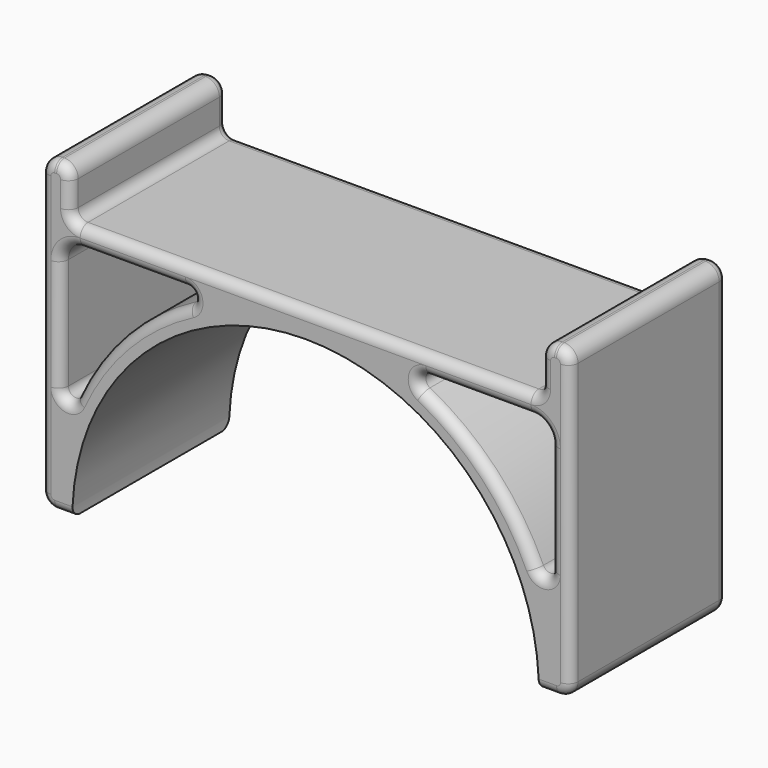
from build123d import *

# Parameters (mm, degrees)
F1_DEPTH = 25.4
F2_R     = 1.778
F3_R     = 2.54
F4_R     = 1.016
F5_R     = 1.27
F6_R     = 1.26999


# Not quite as in the source:
# - a fillet or chamfer is up to 0.001 mm smaller than in the source, because OpenCascade refuses the exact size


with BuildPart() as f1:
    # F0 (on Front) → F1 (new body)
    with BuildSketch(Plane.XZ):
        with BuildLine():
            ThreePointArc((0, 30.226), (21.3730095681, 21.3730095681), (30.226, 0))
            Line((30.226, 0), (34.29, 0))
            Line((34.29, 0), (34.29, 39.878))
            Line((34.29, 39.878), (30.48, 39.878))
            Line((30.48, 39.878), (30.48, 33.528))
            Line((30.48, 33.528), (0, 33.528))
            Line((0, 33.528), (-30.48, 33.528))
            Line((-30.48, 33.528), (-30.48, 39.878))
            Line((-30.48, 39.878), (-34.29, 39.878))
            Line((-34.29, 39.878), (-34.29, 0))
            Line((-34.29, 0), (-30.226, 0))
            ThreePointArc((-30.226, 0), (-21.3730095681, 21.3730095681), (0, 30.226))
        make_face()
        with BuildLine():
            ThreePointArc((-10.6468122929, 30.988), (-24.0911018891, 22.2087722706), (-31.75, 8.0961877449))
            Line((-31.75, 8.0961877449), (-31.75, 30.988))
            Line((-31.75, 30.988), (-10.6468122929, 30.988))
        make_face(mode=Mode.SUBTRACT)
        with BuildLine():
            Line((31.75, 30.988), (31.75, 8.0961877449))
            ThreePointArc((31.75, 8.0961877449), (24.0911018891, 22.2087722706), (10.6468122929, 30.988))
            Line((10.6468122929, 30.988), (31.75, 30.988))
        make_face(mode=Mode.SUBTRACT)
    extrude(amount=F1_DEPTH)

    # F2
    f2_edges = [f1.edges().sort_by_distance(p)[0] for p in [
        (-30.48, -12.7, 39.878),
        (-34.29, -12.7, 39.878),
        (34.29, -12.7, 39.878),
        (30.48, -12.7, 39.878),
        (34.29, -12.7, 0),
        (-34.29, -12.7, 0),
    ]]
    fillet(f2_edges, radius=F2_R)

    # F3
    f3_edges = [f1.edges().sort_by_distance(p)[0] for p in [
        (-31.75, -12.7, 30.988),
        (31.75, -12.7, 30.988),
    ]]
    fillet(f3_edges, radius=F3_R)

    # F4
    f4_edges = [f1.edges().sort_by_distance(p)[0] for p in [
        (-10.646812, -12.7, 30.988),
        (-31.75, -12.7, 8.096188),
        (31.75, -12.7, 8.096188),
        (10.646812, -12.7, 30.988),
    ]]
    fillet(f4_edges, radius=F4_R)

    # F5
    f5_edges = [f1.edges().sort_by_distance(p)[0] for p in [
        (-30.48, -12.7, 33.528),
        (30.48, -12.7, 33.528),
    ]]
    fillet(f5_edges, radius=F5_R)

    # F6 (radius 1.27 in the source; OpenCascade refuses exactly that, so slightly less here)
    f6_edges = [f1.edges().sort_by_distance(p)[0] for p in [
        (-34.29, -25.4, 19.939),
        (-23.757473, -25.4, 22.56531),
        (23.757473, -25.4, 22.56531),
        (0, 0, 33.528),
        (31.75, 0, 21.235504),
        (-23.757473, 0, 22.56531),
    ]]
    fillet(f6_edges, radius=F6_R)


solid = f1.part
